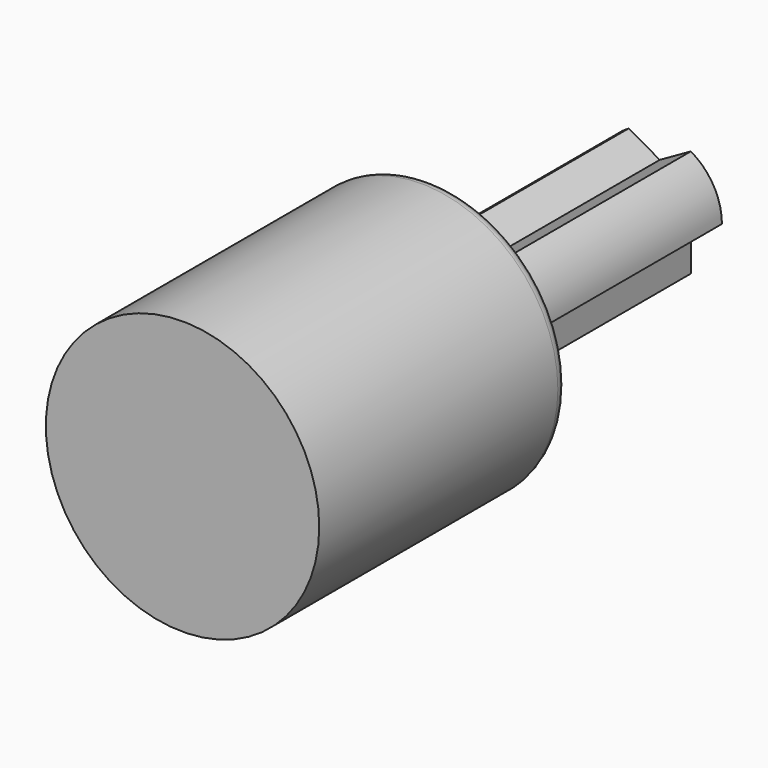
from build123d import *

# Parameters (mm, degrees)
F1_DEPTH = 23
F2_DEPTH = 23
F3_R     = 11
F4_DEPTH = 25
F5_R     = 1


with BuildPart() as f1:
    # F0 (on Front) → F1 (new body)
    with BuildSketch(Plane.XZ):
        Polygon((2.5250660033, -1.4578475367), (5, 0), (2.5, 4.3301270189), (0, 2.9156950735), (-2.5, 4.3301270189), (-5, 0), (-2.5250660033, -1.4578475367), (-2.5, -4.3301270189), (2.5, -4.3301270189), align=None)
    extrude(amount=F1_DEPTH)

    # F0 (on Front) → F2 (join, through all)
    with BuildSketch(Plane.XZ):
        with BuildLine():
            Line((2.5, 4.3301270189), (5, 0))
            ThreePointArc((5, 0), (4.3301270189, 2.5), (2.5, 4.3301270189))
        make_face()
        with BuildLine():
            Line((-5, 0), (-2.5, 4.3301270189))
            ThreePointArc((-2.5, 4.3301270189), (-4.3301270189, 2.5), (-5, 0))
        make_face()
        with BuildLine():
            ThreePointArc((-2.5, -4.3301270189), (0, -5), (2.5, -4.3301270189))
            Line((2.5, -4.3301270189), (-2.5, -4.3301270189))
        make_face()
    extrude(amount=F2_DEPTH)

    # F3 (on face) → F4 (join)
    with BuildSketch(Plane.XZ.offset(23)):
        Circle(F3_R)
        with BuildLine():
            Line((5, 0), (2.5250660033, -1.4578475367))
            Line((2.5250660033, -1.4578475367), (2.5, -4.3301270189))
            ThreePointArc((2.5, -4.3301270189), (0, -5), (-2.5, -4.3301270189))
            Line((-2.5, -4.3301270189), (-2.5250660033, -1.4578475367))
            Line((-2.5250660033, -1.4578475367), (-5, 0))
            ThreePointArc((-5, 0), (-4.3301270189, 2.5), (-2.5, 4.3301270189))
            Line((-2.5, 4.3301270189), (0, 2.9156950735))
            Line((0, 2.9156950735), (2.5, 4.3301270189))
            ThreePointArc((2.5, 4.3301270189), (4.3301270189, 2.5), (5, 0))
        make_face(mode=Mode.SUBTRACT)
        with BuildLine():
            Line((2.5, -4.3301270189), (2.5250660033, -1.4578475367))
            Line((2.5250660033, -1.4578475367), (5, 0))
            ThreePointArc((5, 0), (4.3301270189, 2.5), (2.5, 4.3301270189))
            Line((2.5, 4.3301270189), (0, 2.9156950735))
            Line((0, 2.9156950735), (-2.5, 4.3301270189))
            ThreePointArc((-2.5, 4.3301270189), (-4.3301270189, 2.5), (-5, 0))
            Line((-5, 0), (-2.5250660033, -1.4578475367))
            Line((-2.5250660033, -1.4578475367), (-2.5, -4.3301270189))
            ThreePointArc((-2.5, -4.3301270189), (0, -5), (2.5, -4.3301270189))
        make_face()
    extrude(amount=F4_DEPTH)

    # F5
    f5_edges = [f1.edges().sort_by_distance(p)[0] for p in [
        (-11, -23, 0),
        (3.762533, -23, -0.728924),
        (4.330127, -23, 2.5),
        (1.25, -23, 3.622911),
        (-1.25, -23, 3.622911),
        (-4.330127, -23, 2.5),
        (-3.762533, -23, -0.728924),
        (-2.512533, -23, -2.893987),
        (0, -23, -5),
        (2.512533, -23, -2.893987),
    ]]
    fillet(f5_edges, radius=F5_R)


solid = f1.part
